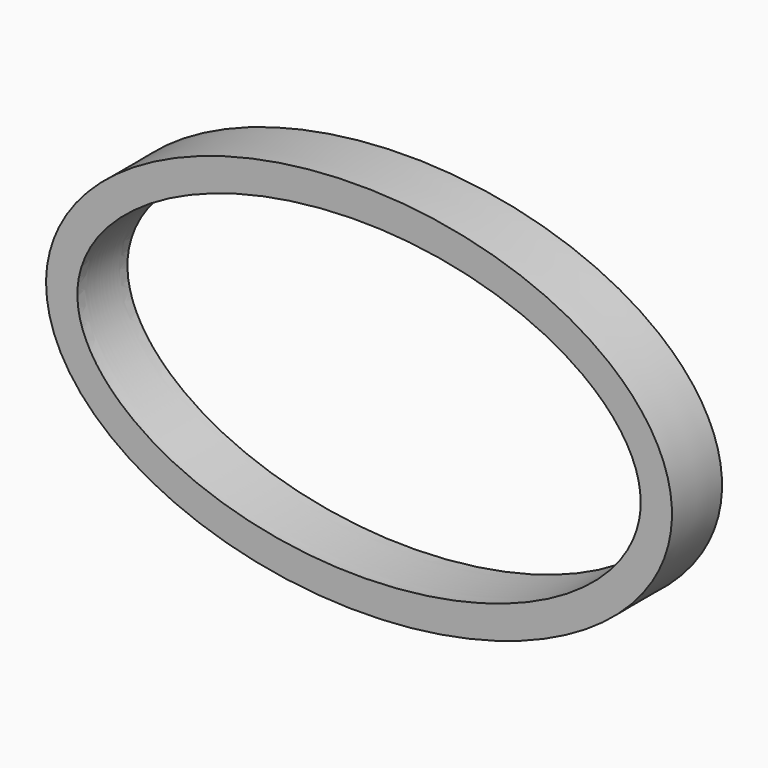
from build123d import *

# Parameters (mm, degrees)
F1_DEPTH = 12.7


# Not quite as in the source:
# - the dataset's text gives a spline's control points without its knots; the knots are read off the source's solid


with BuildPart() as f1:
    # F0 (on Front) → F1 (new body)
    with BuildSketch(Plane.XZ):
        with BuildLine():
            add(Edge.make_bspline(
                [(63.5, 20.9593381733), (63.5, 59.0593381733), (0, 59.0593381733), (-63.5, 59.0593381733), (-63.5, 20.9593381733)],
                knots=[0, 0, 0, 1.5707963268, 1.5707963268, 3.1415926536, 3.1415926536, 3.1415926536], degree=2, weights=[1, 0.7071067812, 1, 0.7071067812, 1]))
            add(Edge.make_bspline(
                [(-63.5, 20.9593381733), (-63.5, -17.1406618267), (0, -17.1406618267), (63.5, -17.1406618267), (63.5, 20.9593381733)],
                knots=[3.1415926536, 3.1415926536, 3.1415926536, 4.7123889804, 4.7123889804, 6.2831853072, 6.2831853072, 6.2831853072], degree=2, weights=[1, 0.7071067812, 1, 0.7071067812, 1]))
        make_face()
        with BuildLine():
            add(Edge.make_bspline(
                [(-57.1500017911, 20.9593381733), (-57.1500017911, 20.5037470944), (-57.1122902213, 19.5925649367), (-56.8869841088, 17.7768493493), (-56.3227681021, 15.5026509765), (-55.1736964536, 12.7511242731), (-53.5267765887, 9.984666464), (-51.362414901, 7.2305016893), (-48.6714850573, 4.5265238967), (-45.9900495115, 2.3493864122), (-43.5867796933, 0.6747992402), (-41.6535307679, -0.5445851955), (-39.6044981147, -1.7145683435), (-36.7426493863, -3.1937696987), (-32.9269482144, -4.8886439263), (-28.0132867087, -6.6526895833), (-22.8094881511, -8.1286312373), (-17.3614595644, -9.2999739711), (-11.715301465, -10.1522960471), (-6.8823620796, -10.5859661799), (-2.9639604007, -10.7611786742), (0, -10.8054060896), (2.9639604007, -10.7611786742), (6.8823620796, -10.5859661799), (11.715301465, -10.1522960471), (17.3614595644, -9.2999739711), (22.8094881511, -8.1286312373), (28.0132867087, -6.6526895833), (32.9269482144, -4.8886439263), (36.7426493863, -3.1937696987), (39.6044981147, -1.7145683435), (41.6535307679, -0.5445851955), (43.5867796933, 0.6747992402), (45.9900495115, 2.3493864122), (48.6714850573, 4.5265238967), (51.362414901, 7.2305016893), (53.5267765887, 9.984666464), (55.1736964536, 12.7511242731), (56.3227681021, 15.5026509765), (56.8869841088, 17.7768493493), (57.1122902213, 19.5925649367), (57.1500017911, 20.5037470944), (57.1500017911, 20.9593381733)],
                knots=[0.5, 0.5, 0.5, 0.5, 0.5078125, 0.515625, 0.53125, 0.546875, 0.5625, 0.578125, 0.59375, 0.609375, 0.6171875, 0.625, 0.6328125, 0.640625, 0.65625, 0.671875, 0.6875, 0.703125, 0.71875, 0.734375, 0.7421875, 0.75, 0.7578125, 0.765625, 0.78125, 0.796875, 0.8125, 0.828125, 0.84375, 0.859375, 0.8671875, 0.875, 0.8828125, 0.890625, 0.90625, 0.921875, 0.9375, 0.953125, 0.96875, 0.984375, 0.9921875, 1, 1, 1, 1], degree=3))
            add(Edge.make_bspline(
                [(57.1500017911, 20.9593381733), (57.1500017911, 21.4149292521), (57.1122902213, 22.3261114098), (56.8869841088, 24.1418269973), (56.3227681021, 26.4160253701), (55.1736964536, 29.1675520735), (53.5267765887, 31.9340098826), (51.362414901, 34.6881746572), (48.6714850573, 37.3921524499), (45.9900495115, 39.5692899343), (43.5867796933, 41.2438771063), (41.6535307679, 42.463261542), (39.6044981147, 43.6332446901), (36.7426493863, 45.1124460453), (32.9269482144, 46.8073202728), (28.0132867087, 48.5713659298), (22.8094881511, 50.0473075839), (17.3614595644, 51.2186503177), (11.715301465, 52.0709723936), (6.8823620796, 52.5046425265), (2.9639604007, 52.6798550208), (0, 52.7240824362), (-2.9639604007, 52.6798550208), (-6.8823620796, 52.5046425265), (-11.715301465, 52.0709723936), (-17.3614595644, 51.2186503177), (-22.8094881511, 50.0473075839), (-28.0132867087, 48.5713659298), (-32.9269482144, 46.8073202728), (-36.7426493863, 45.1124460453), (-39.6044981147, 43.6332446901), (-41.6535307679, 42.463261542), (-43.5867796933, 41.2438771063), (-45.9900495115, 39.5692899343), (-48.6714850573, 37.3921524499), (-51.362414901, 34.6881746572), (-53.5267765887, 31.9340098826), (-55.1736964536, 29.1675520735), (-56.3227681021, 26.4160253701), (-56.8869841088, 24.1418269973), (-57.1122902213, 22.3261114098), (-57.1500017911, 21.4149292521), (-57.1500017911, 20.9593381733)],
                knots=[0, 0, 0, 0, 0.0078125, 0.015625, 0.03125, 0.046875, 0.0625, 0.078125, 0.09375, 0.109375, 0.1171875, 0.125, 0.1328125, 0.140625, 0.15625, 0.171875, 0.1875, 0.203125, 0.21875, 0.234375, 0.2421875, 0.25, 0.2578125, 0.265625, 0.28125, 0.296875, 0.3125, 0.328125, 0.34375, 0.359375, 0.3671875, 0.375, 0.3828125, 0.390625, 0.40625, 0.421875, 0.4375, 0.453125, 0.46875, 0.484375, 0.4921875, 0.5, 0.5, 0.5, 0.5], degree=3))
        make_face(mode=Mode.SUBTRACT)
    extrude(amount=F1_DEPTH)


solid = f1.part
